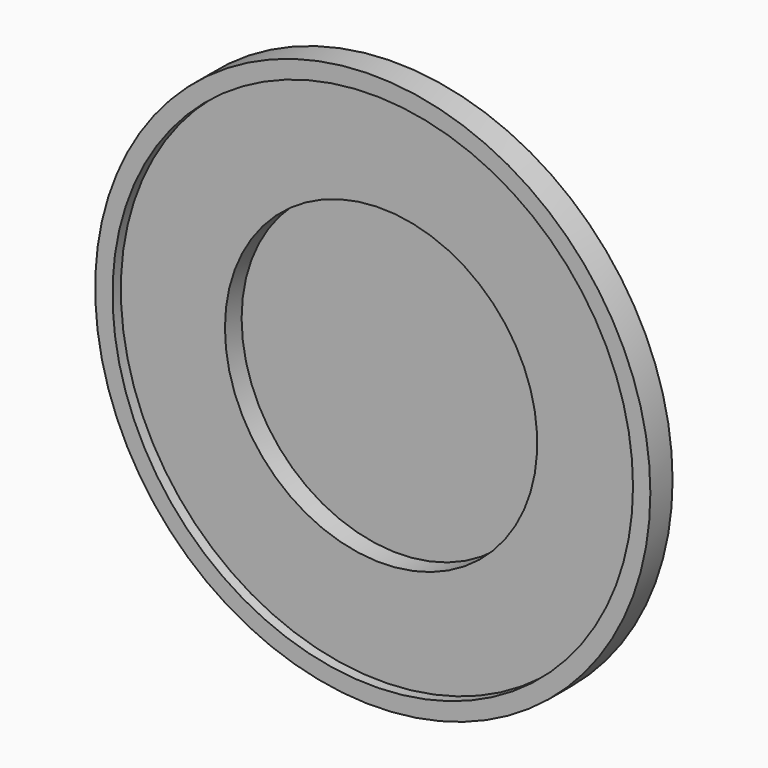
from build123d import *

# Parameters (mm, degrees)
F0_R     = 40
F1_DEPTH = 3
F2_DEPTH = 1
F3_R     = 25
F4_DEPTH = 3
F5_T     = -2.5


with BuildPart() as f1:
    # F0 (on Front) → F1 (new body)
    with BuildSketch(Plane.XZ):
        Circle(F0_R)
    extrude(amount=F1_DEPTH)

    # F2 (add): a face of the model
    f2_faces = [f1.faces().sort_by_distance(p)[0] for p in [
        (0, -3, 0),
    ]]
    extrude(f2_faces, amount=F2_DEPTH)

    # F3 (on face) → F4 (join)
    with BuildSketch(Plane(origin=(0, 0, 0), x_dir=(-1, 0, 0), z_dir=(0, 1, 0))):
        Circle(F3_R)
    extrude(amount=F4_DEPTH)

    # F5
    f5_openings = [f1.faces().sort_by_distance(p)[0] for p in [
        (0, -4, 0),
    ]]
    offset(amount=F5_T, openings=f5_openings, kind=Kind.INTERSECTION)


solid = f1.part
